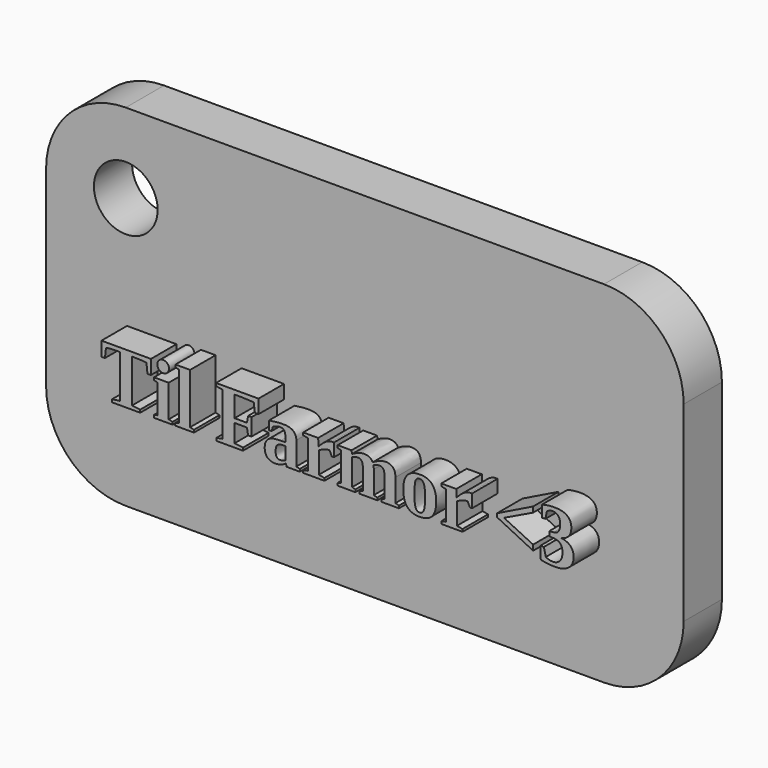
from build123d import *

# Parameters (mm, degrees)
F1_DEPTH     = 3
F2_R         = 2
F3_DEPTH     = 25
F4_TEXT_SIZE = 4.8761904762
F5_DEPTH     = 2


# Not quite as in the source:
# - Text() gives the source's letters only with a copy of the font that has no kerning and outlines rounded to 1/6400 em; it was checked with that copy


with BuildPart() as f1:
    # F0 (on Front) → F1 (new body)
    with BuildSketch(Plane.XZ):
        with BuildLine():
            ThreePointArc((0, 5), (1.4644660941, 1.4644660941), (5, 0))
            Line((5, 0), (35, 0))
            ThreePointArc((35, 0), (38.5355339059, 1.4644660941), (40, 5))
            Line((40, 5), (40, 17))
            ThreePointArc((40, 17), (38.5355339059, 20.5355339059), (35, 22))
            Line((35, 22), (5, 22))
            ThreePointArc((5, 22), (1.4644660941, 20.5355339059), (0, 17))
            Line((0, 17), (0, 5))
        make_face()
    extrude(amount=F1_DEPTH)

    # F2 (on face) → F3 (cut)
    with BuildSketch(Plane.XZ.offset(3)):
        with Locations((5, 17)):
            Circle(F2_R)
    extrude(amount=-F3_DEPTH, mode=Mode.SUBTRACT)

    # F4 (on face) → F5 (join)
    with BuildSketch(Plane.XZ.offset(3)):
        with Locations((5, 6.7719344919)):
            Text('Til Farmor <3', F4_TEXT_SIZE, font='Tinos', font_style=FontStyle.BOLD, text_align=(TextAlign.LEFT, TextAlign.BOTTOM))
    extrude(amount=F5_DEPTH)


solid = f1.part
